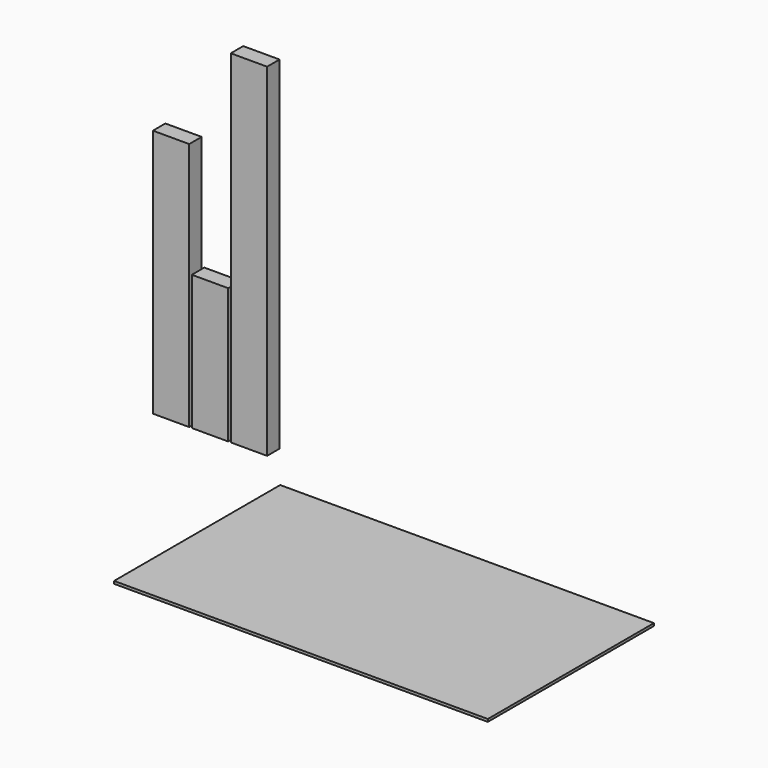
from build123d import *

# Parameters (mm, degrees)
F4_W     = 88.9
F4_H     = 38.1
F5_DEPTH = 609.6
F6_DEPTH = 330.2
F7_DEPTH = 838.2
F8_W     = 914.4
F8_H     = 508
F9_DEPTH = 6.35


# Not quite as in the source:
# - a length typed as a fraction of an inch, garbled in the dataset ("3 / 203.2 mm" for 3/8 in), is restored


with BuildPart() as f5:
    # F4 (on Top) → F5 (new body)
    with BuildSketch(Plane.XY):
        with Locations((-126.334846382, 34.7348225479)):
            Rectangle(F4_W, F4_H)
    extrude(amount=F5_DEPTH)


with BuildPart() as f6:
    # F4 (on Top) → F6 (new body)
    with BuildSketch(Plane.XY):
        with Locations((-31.084846382, 34.7348225479)):
            Rectangle(F4_W, F4_H)
    extrude(amount=F6_DEPTH)


with BuildPart() as f7:
    # F4 (on Top) → F7 (new body)
    with BuildSketch(Plane.XY):
        with Locations((64.165153618, 34.7348225479)):
            Rectangle(F4_W, F4_H)
    extrude(amount=F7_DEPTH)


with BuildPart() as f9:
    # F8 (on Top) → F9 (new body)
    with BuildSketch(Plane.XY):
        with Locations((668.3245897293, -326.4362514019)):
            Rectangle(F8_W, F8_H)
    extrude(amount=F9_DEPTH)


solid = Compound([f5.part, f6.part, f7.part, f9.part])
